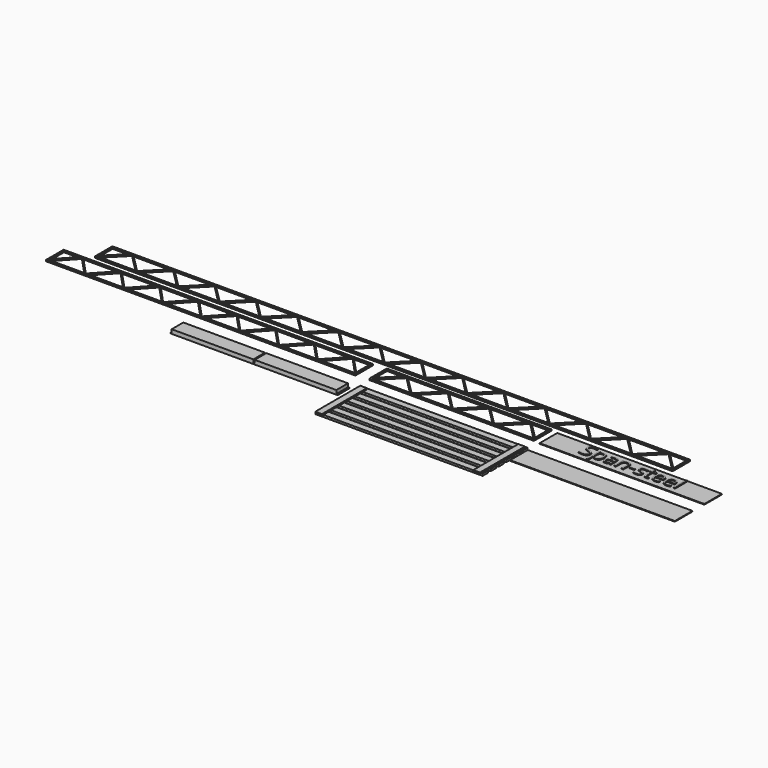
from build123d import *

# Parameters (mm, degrees)
F1_DEPTH     = 0.508
F2_W         = 63.246
F2_H         = 8.4328
F3_DEPTH     = 0.508
F5_DEPTH     = 0.508
F6_W         = 63.246
F6_H         = 8.4328
F6_W_2       = 1.8878322943
F6_H_2       = 0.5845634549
F6_W_3       = 0.6387124907
F6_H_3       = 5.9846991182
F6_TEXT_SIZE = 7.8762233922
F7_DEPTH     = 0.254
F8_DEPTH     = 0.508
F9_W         = 2.54
F9_H         = 1.905
F10_DEPTH    = 0.762
F9_W_2       = 58.166
F9_H_2       = 2.54
F9_W_3       = 0.508
F9_H_3       = 1.27
F9_H_4       = 0.635
F11_DEPTH    = 0.508
F12_W        = 0.508
F12_H        = 5.588
F12_W_2      = 31.369
F13_DEPTH    = 0.254
F14_DEPTH    = 1.58496


# Not quite as in the source:
# - Text() gives the source's letters only with a copy of the font that has no kerning and outlines rounded to 1/6400 em; it was checked with that copy


with BuildPart() as f1:
    # F0 (on Top) → F1 (new body)
    with BuildSketch(Plane.XY):
        Polygon((-113.8428, 0), (-2.8956, 0), (108.0516, 0), (108.0516, 8.4328), (-2.8956, 8.4328), (-113.8428, 8.4328), align=None)
        Polygon((-113.3348, 1.016), (-113.3348, 7.9248), (-106.426, 7.9248), align=None, mode=Mode.SUBTRACT)
        Polygon((-98.5012, 0.508), (-113.3348, 0.508), (-105.918, 7.9248), align=None, mode=Mode.SUBTRACT)
        Polygon((-90.5764, 7.9248), (-97.9932, 0.508), (-105.41, 7.9248), align=None, mode=Mode.SUBTRACT)
        Polygon((-82.6516, 0.508), (-97.4852, 0.508), (-90.0684, 7.9248), align=None, mode=Mode.SUBTRACT)
        Polygon((-74.7268, 7.9248), (-82.1436, 0.508), (-89.5604, 7.9248), align=None, mode=Mode.SUBTRACT)
        Polygon((-66.802, 0.508), (-81.6356, 0.508), (-74.2188, 7.9248), align=None, mode=Mode.SUBTRACT)
        Polygon((-58.8772, 7.9248), (-66.294, 0.508), (-73.7108, 7.9248), align=None, mode=Mode.SUBTRACT)
        Polygon((-50.9524, 0.508), (-65.786, 0.508), (-58.3692, 7.9248), align=None, mode=Mode.SUBTRACT)
        Polygon((-43.0276, 7.9248), (-50.4444, 0.508), (-57.8612, 7.9248), align=None, mode=Mode.SUBTRACT)
        Polygon((-35.1028, 0.508), (-49.9364, 0.508), (-42.5196, 7.9248), align=None, mode=Mode.SUBTRACT)
        Polygon((-27.178, 7.9248), (-34.5948, 0.508), (-42.0116, 7.9248), align=None, mode=Mode.SUBTRACT)
        Polygon((-19.2532, 0.508), (-34.0868, 0.508), (-26.67, 7.9248), align=None, mode=Mode.SUBTRACT)
        Polygon((-11.3284, 7.9248), (-18.7452, 0.508), (-26.162, 7.9248), align=None, mode=Mode.SUBTRACT)
        Polygon((-3.4036, 0.508), (-18.2372, 0.508), (-10.8204, 7.9248), align=None, mode=Mode.SUBTRACT)
        Polygon((-10.3124, 7.9248), (-2.8956, 7.9248), (4.5212, 7.9248), (-2.8956, 0.508), align=None, mode=Mode.SUBTRACT)
        Polygon((5.0292, 7.9248), (12.446, 0.508), (-2.3876, 0.508), align=None, mode=Mode.SUBTRACT)
        Polygon((20.3708, 7.9248), (12.954, 0.508), (5.5372, 7.9248), align=None, mode=Mode.SUBTRACT)
        Polygon((20.8788, 7.9248), (28.2956, 0.508), (13.462, 0.508), align=None, mode=Mode.SUBTRACT)
        Polygon((21.3868, 7.9248), (36.2204, 7.9248), (28.8036, 0.508), align=None, mode=Mode.SUBTRACT)
        Polygon((36.7284, 7.9248), (44.1452, 0.508), (29.3116, 0.508), align=None, mode=Mode.SUBTRACT)
        Polygon((52.07, 7.9248), (44.6532, 0.508), (37.2364, 7.9248), align=None, mode=Mode.SUBTRACT)
        Polygon((52.578, 7.9248), (59.9948, 0.508), (45.1612, 0.508), align=None, mode=Mode.SUBTRACT)
        Polygon((67.9196, 7.9248), (60.5028, 0.508), (53.086, 7.9248), align=None, mode=Mode.SUBTRACT)
        Polygon((75.8444, 0.508), (61.0108, 0.508), (68.4276, 7.9248), align=None, mode=Mode.SUBTRACT)
        Polygon((68.9356, 7.9248), (83.7692, 7.9248), (76.3524, 0.508), align=None, mode=Mode.SUBTRACT)
        Polygon((84.2772, 7.9248), (91.694, 0.508), (76.8604, 0.508), align=None, mode=Mode.SUBTRACT)
        Polygon((84.7852, 7.9248), (99.6188, 7.9248), (92.202, 0.508), align=None, mode=Mode.SUBTRACT)
        Polygon((100.1268, 7.9248), (107.5436, 0.508), (92.71, 0.508), align=None, mode=Mode.SUBTRACT)
        Polygon((100.6348, 7.9248), (107.5436, 7.9248), (107.5436, 1.016), align=None, mode=Mode.SUBTRACT)
    extrude(amount=F1_DEPTH)


with BuildPart() as f3:
    # F2 (on Top) → F3 (new body)
    with BuildSketch(Plane.XY):
        with Locations((31.623, -6.3287943188)):
            Rectangle(F2_W, F2_H)
        Polygon((0.508, -9.5291943188), (0.508, -2.6203943188), (7.4168, -2.6203943188), align=None, mode=Mode.SUBTRACT)
        Polygon((15.3416, -10.0371943188), (0.508, -10.0371943188), (7.9248, -2.6203943188), align=None, mode=Mode.SUBTRACT)
        Polygon((23.2664, -2.6203943188), (15.8496, -10.0371943188), (8.4328, -2.6203943188), align=None, mode=Mode.SUBTRACT)
        Polygon((31.1912, -10.0371943188), (16.3576, -10.0371943188), (23.7744, -2.6203943188), align=None, mode=Mode.SUBTRACT)
        Polygon((39.116, -2.6203943188), (31.6992, -10.0371943188), (24.2824, -2.6203943188), align=None, mode=Mode.SUBTRACT)
        Polygon((47.0408, -10.0371943188), (32.2072, -10.0371943188), (39.624, -2.6203943188), align=None, mode=Mode.SUBTRACT)
        Polygon((47.5488, -10.0371943188), (40.132, -2.6203943188), (54.9656, -2.6203943188), align=None, mode=Mode.SUBTRACT)
        Polygon((62.738, -10.0371943188), (48.0568, -10.0371943188), (55.4736, -2.6203943188), align=None, mode=Mode.SUBTRACT)
        Polygon((55.9816, -2.6203943188), (62.738, -2.6203943188), (62.738, -9.3767943188), align=None, mode=Mode.SUBTRACT)
    extrude(amount=F3_DEPTH)


with BuildPart() as f5:
    # F4 (on Top) → F5 (new body)
    with BuildSketch(Plane.XY):
        Polygon((-5.08, -10.8726160142), (-5.08, -2.4398160142), (-123.3604462539, -2.4398160142), (-123.8684462539, -2.4398160142), (-123.8684462539, -10.8726160142), (-123.3604462539, -10.8726160142), align=None)
        Polygon((-116.444168363, -2.9478160142), (-109.5278904721, -10.3646160142), (-123.3604462539, -10.3646160142), align=None, mode=Mode.SUBTRACT)
        Polygon((-101.5956125813, -2.9478160142), (-94.6793346904, -10.3646160142), (-108.5118904721, -10.3646160142), align=None, mode=Mode.SUBTRACT)
        Polygon((-86.7470567995, -2.9478160142), (-79.8307789087, -10.3646160142), (-93.6633346904, -10.3646160142), align=None, mode=Mode.SUBTRACT)
        Polygon((-57.0499452361, -2.9478160142), (-50.1336673452, -10.3646160142), (-63.9662231269, -10.3646160142), align=None, mode=Mode.SUBTRACT)
        Polygon((-42.2013894543, -2.9478160142), (-35.2851115635, -10.3646160142), (-49.1176673452, -10.3646160142), align=None, mode=Mode.SUBTRACT)
        Polygon((-116.9555484155, -2.9478160142), (-123.3604462539, -9.8195863482), (-123.3604462539, -2.9478160142), align=None, mode=Mode.SUBTRACT)
        Polygon((-108.4620648578, -9.7664212797), (-109.0198904721, -10.3646160142), (-115.9327883105, -2.9478160142), (-102.1069926338, -2.9478160142), align=None, mode=Mode.SUBTRACT)
        Polygon((-87.258436852, -2.9478160142), (-94.1713346904, -10.3646160142), (-94.7291603047, -9.7664212797), (-101.0842325287, -2.9478160142), align=None, mode=Mode.SUBTRACT)
        Polygon((-86.235676747, -2.9478160142), (-72.4098810703, -2.9478160142), (-79.3227789087, -10.3646160142), align=None, mode=Mode.SUBTRACT)
        Polygon((-71.8985010178, -2.9478160142), (-64.9822231269, -10.3646160142), (-78.8147789087, -10.3646160142), align=None, mode=Mode.SUBTRACT)
        Polygon((-57.5613252886, -2.9478160142), (-64.4742231269, -10.3646160142), (-71.3871209653, -2.9478160142), align=None, mode=Mode.SUBTRACT)
        Polygon((-56.5385651835, -2.9478160142), (-42.7127695068, -2.9478160142), (-49.0678417309, -9.7664212797), (-49.6256673452, -10.3646160142), align=None, mode=Mode.SUBTRACT)
        Polygon((-41.6900094018, -2.9478160142), (-27.8642137251, -2.9478160142), (-34.7771115635, -10.3646160142), (-35.3349371778, -9.7664212797), align=None, mode=Mode.SUBTRACT)
        Polygon((-27.3528336726, -2.9478160142), (-20.4365557817, -10.3646160142), (-34.2691115635, -10.3646160142), align=None, mode=Mode.SUBTRACT)
        Polygon((-26.8414536201, -2.9478160142), (-13.0156579434, -2.9478160142), (-19.3707301674, -9.7664212797), (-19.9285557817, -10.3646160142), align=None, mode=Mode.SUBTRACT)
        Polygon((-12.5042778909, -2.9478160142), (-5.588, -10.3646160142), (-19.4205557817, -10.3646160142), align=None, mode=Mode.SUBTRACT)
        Polygon((-11.9928978384, -2.9478160142), (-5.588, -2.9478160142), (-5.588, -9.8566160142), align=None, mode=Mode.SUBTRACT)
    extrude(amount=F5_DEPTH)


with BuildPart() as f7:
    # F6 (on Top) → F7 (new body)
    with BuildSketch(Plane.XY):
        with Locations((97.409, -6.7564)):
            Rectangle(F6_W, F6_H)
        with BuildLine():
            add(Edge.make_bspline(
                [(81.9722174812, -6.2846355502), (82.3044956555, -6.6464495623), (82.3044956555, -7.2223983979)],
                knots=[0, 0, 0, 1, 1, 1], degree=2))
            add(Edge.make_bspline(
                [(82.3044956555, -7.2223983979), (82.3044956555, -7.9644863206), (81.7660819471, -8.3804493685)],
                knots=[0, 0, 0, 1, 1, 1], degree=2))
            add(Edge.make_bspline(
                [(81.7660819471, -8.3804493685), (81.2276682386, -8.7964124164), (80.3046733099, -8.7964124164)],
                knots=[0, 0, 0, 1, 1, 1], degree=2))
            add(Edge.make_bspline(
                [(80.3046733099, -8.7964124164), (79.305377467, -8.7964124164), (78.7663484286, -8.5379738364)],
                knots=[0, 0, 0, 1, 1, 1], degree=2))
            Line((78.7663484286, -8.5379738364), (78.7663484286, -7.907875965))
            add(Edge.make_bspline(
                [(78.7663484286, -7.907875965), (79.1133945218, -8.0530938338), (79.5207429504, -8.1380093672)],
                knots=[0, 0, 0, 1, 1, 1], degree=2))
            add(Edge.make_bspline(
                [(79.5207429504, -8.1380093672), (79.9280913789, -8.2229249007), (80.3280558481, -8.2229249007)],
                knots=[0, 0, 0, 1, 1, 1], degree=2))
            add(Edge.make_bspline(
                [(80.3280558481, -8.2229249007), (80.9815362576, -8.2229249007), (81.3125837721, -7.9749469298)],
                knots=[0, 0, 0, 1, 1, 1], degree=2))
            add(Edge.make_bspline(
                [(81.3125837721, -7.9749469298), (81.6436312865, -7.7269689589), (81.6436312865, -7.2839313931)],
                knots=[0, 0, 0, 1, 1, 1], degree=2))
            add(Edge.make_bspline(
                [(81.6436312865, -7.2839313931), (81.6436312865, -6.9922649956), (81.5261032656, -6.80582002)],
                knots=[0, 0, 0, 1, 1, 1], degree=2))
            add(Edge.make_bspline(
                [(81.5261032656, -6.80582002), (81.4085752447, -6.6193750444), (81.1335227559, -6.4612352466)],
                knots=[0, 0, 0, 1, 1, 1], degree=2))
            add(Edge.make_bspline(
                [(81.1335227559, -6.4612352466), (80.8584702671, -6.3030954488), (80.2972893504, -6.1037285442)],
                knots=[0, 0, 0, 1, 1, 1], degree=2))
            add(Edge.make_bspline(
                [(80.2972893504, -6.1037285442), (79.5133589909, -5.8231380859), (79.1767735069, -5.4385568655)],
                knots=[0, 0, 0, 1, 1, 1], degree=2))
            add(Edge.make_bspline(
                [(79.1767735069, -5.4385568655), (78.8401880229, -5.0539756452), (78.8401880229, -4.434953713)],
                knots=[0, 0, 0, 1, 1, 1], degree=2))
            add(Edge.make_bspline(
                [(78.8401880229, -4.434953713), (78.8401880229, -3.7851652831), (79.3281446752, -3.4005840628)],
                knots=[0, 0, 0, 1, 1, 1], degree=2))
            add(Edge.make_bspline(
                [(79.3281446752, -3.4005840628), (79.8161013276, -3.0160028425), (80.6209529055, -3.0160028425)],
                knots=[0, 0, 0, 1, 1, 1], degree=2))
            add(Edge.make_bspline(
                [(80.6209529055, -3.0160028425), (81.4590323008, -3.0160028425), (82.1629697665, -3.3236678187)],
                knots=[0, 0, 0, 1, 1, 1], degree=2))
            Line((82.1629697665, -3.3236678187), (81.9586802222, -3.8922326949))
            add(Edge.make_bspline(
                [(81.9586802222, -3.8922326949), (81.262126716, -3.6005662974), (80.6049543267, -3.6005662974)],
                knots=[0, 0, 0, 1, 1, 1], degree=2))
            add(Edge.make_bspline(
                [(80.6049543267, -3.6005662974), (80.0856158468, -3.6005662974), (79.7933341193, -3.8233157402)],
                knots=[0, 0, 0, 1, 1, 1], degree=2))
            add(Edge.make_bspline(
                [(79.7933341193, -3.8233157402), (79.5010523919, -4.046065183), (79.5010523919, -4.4423376724)],
                knots=[0, 0, 0, 1, 1, 1], degree=2))
            add(Edge.make_bspline(
                [(79.5010523919, -4.4423376724), (79.5010523919, -4.7340040699), (79.6087351336, -4.9210643755)],
                knots=[0, 0, 0, 1, 1, 1], degree=2))
            add(Edge.make_bspline(
                [(79.6087351336, -4.9210643755), (79.7164178753, -5.108124681), (79.9723951355, -5.263803159)],
                knots=[0, 0, 0, 1, 1, 1], degree=2))
            add(Edge.make_bspline(
                [(79.9723951355, -5.263803159), (80.2283723957, -5.419481637), (80.7550948351, -5.6077726025)],
                knots=[0, 0, 0, 1, 1, 1], degree=2))
            add(Edge.make_bspline(
                [(80.7550948351, -5.6077726025), (81.6399393068, -5.9228215382), (81.9722174812, -6.2846355502)],
                knots=[0, 0, 0, 1, 1, 1], degree=2))
        make_face(mode=Mode.SUBTRACT)
        with BuildLine():
            add(Edge.make_bspline(
                [(86.6074980135, -8.2210789108), (86.1441545593, -8.7964124164), (85.3208430828, -8.7964124164)],
                knots=[0, 0, 0, 1, 1, 1], degree=2))
            add(Edge.make_bspline(
                [(85.3208430828, -8.7964124164), (84.9085720146, -8.7964124164), (84.5682945509, -8.6444259181)],
                knots=[0, 0, 0, 1, 1, 1], degree=2))
            add(Edge.make_bspline(
                [(84.5682945509, -8.6444259181), (84.2280170871, -8.4924394199), (83.9978836849, -8.1761598243)],
                knots=[0, 0, 0, 1, 1, 1], degree=2))
            Line((83.9978836849, -8.1761598243), (83.9511186085, -8.1761598243))
            add(Edge.make_bspline(
                [(83.9511186085, -8.1761598243), (83.9978836849, -8.5453577958), (83.9978836849, -8.8764053102)],
                knots=[0, 0, 0, 1, 1, 1], degree=2))
            Line((83.9978836849, -8.8764053102), (83.9978836849, -10.6116357763))
            Line((83.9978836849, -10.6116357763), (83.3591711942, -10.6116357763))
            Line((83.3591711942, -10.6116357763), (83.3591711942, -4.5038706677))
            Line((83.3591711942, -4.5038706677), (83.8785096741, -4.5038706677))
            Line((83.8785096741, -4.5038706677), (83.9671171872, -5.0810501631))
            Line((83.9671171872, -5.0810501631), (83.9978836849, -5.0810501631))
            add(Edge.make_bspline(
                [(83.9978836849, -5.0810501631), (84.2440156659, -4.7340040699), (84.5707558707, -4.5801715818)],
                knots=[0, 0, 0, 1, 1, 1], degree=2))
            add(Edge.make_bspline(
                [(84.5707558707, -4.5801715818), (84.8974960755, -4.4263390936), (85.3208430828, -4.4263390936)],
                knots=[0, 0, 0, 1, 1, 1], degree=2))
            add(Edge.make_bspline(
                [(85.3208430828, -4.4263390936), (86.1589224781, -4.4263390936), (86.6148819729, -4.9998266094)],
                knots=[0, 0, 0, 1, 1, 1], degree=2))
            add(Edge.make_bspline(
                [(86.6148819729, -4.9998266094), (87.0708414677, -5.5733141251), (87.0708414677, -6.6070684454)],
                knots=[0, 0, 0, 1, 1, 1], degree=2))
            add(Edge.make_bspline(
                [(87.0708414677, -6.6070684454), (87.0708414677, -7.6457454052), (86.6074980135, -8.2210789108)],
                knots=[0, 0, 0, 1, 1, 1], degree=2))
        make_face(mode=Mode.SUBTRACT)
        with BuildLine():
            Line((91.2513931652, -8.7188808424), (90.7775891017, -8.7188808424))
            Line((90.7775891017, -8.7188808424), (90.6508311315, -8.1183188087))
            Line((90.6508311315, -8.1183188087), (90.6200646339, -8.1183188087))
            add(Edge.make_bspline(
                [(90.6200646339, -8.1183188087), (90.3050156982, -8.5145912982), (89.9918127523, -8.6555018573)],
                knots=[0, 0, 0, 1, 1, 1], degree=2))
            add(Edge.make_bspline(
                [(89.9918127523, -8.6555018573), (89.6786098065, -8.7964124164), (89.2084977228, -8.7964124164)],
                knots=[0, 0, 0, 1, 1, 1], degree=2))
            add(Edge.make_bspline(
                [(89.2084977228, -8.7964124164), (88.5820918311, -8.7964124164), (88.2264311186, -8.4727488614)],
                knots=[0, 0, 0, 1, 1, 1], degree=2))
            add(Edge.make_bspline(
                [(88.2264311186, -8.4727488614), (87.870770406, -8.1490853064), (87.870770406, -7.5534459123)],
                knots=[0, 0, 0, 1, 1, 1], degree=2))
            add(Edge.make_bspline(
                [(87.870770406, -7.5534459123), (87.870770406, -6.2772515908), (89.9124351885, -6.2157185956)],
                knots=[0, 0, 0, 1, 1, 1], degree=2))
            Line((89.9124351885, -6.2157185956), (90.6274485933, -6.1923360574))
            Line((90.6274485933, -6.1923360574), (90.6274485933, -5.9302054976))
            add(Edge.make_bspline(
                [(90.6274485933, -5.9302054976), (90.6274485933, -5.4342495559), (90.4145444297, -5.1979628541)],
                knots=[0, 0, 0, 1, 1, 1], degree=2))
            add(Edge.make_bspline(
                [(90.4145444297, -5.1979628541), (90.2016402662, -4.9616761523), (89.7315281824, -4.9616761523)],
                knots=[0, 0, 0, 1, 1, 1], degree=2))
            add(Edge.make_bspline(
                [(89.7315281824, -4.9616761523), (89.2048057431, -4.9616761523), (88.5402493944, -5.2841090474)],
                knots=[0, 0, 0, 1, 1, 1], degree=2))
            Line((88.5402493944, -5.2841090474), (88.3433438096, -4.7955370652))
            add(Edge.make_bspline(
                [(88.3433438096, -4.7955370652), (88.6547007655, -4.6269366582), (89.0257447269, -4.5309451856)],
                knots=[0, 0, 0, 1, 1, 1], degree=2))
            add(Edge.make_bspline(
                [(89.0257447269, -4.5309451856), (89.3967886883, -4.434953713), (89.7709092994, -4.434953713)],
                knots=[0, 0, 0, 1, 1, 1], degree=2))
            add(Edge.make_bspline(
                [(89.7709092994, -4.434953713), (90.5240731613, -4.434953713), (90.8877331632, -4.7690778772)],
                knots=[0, 0, 0, 1, 1, 1], degree=2))
            add(Edge.make_bspline(
                [(90.8877331632, -4.7690778772), (91.2513931652, -5.1032020414), (91.2513931652, -5.8415979844)],
                knots=[0, 0, 0, 1, 1, 1], degree=2))
            Line((91.2513931652, -5.8415979844), (91.2513931652, -8.7188808424))
        make_face(mode=Mode.SUBTRACT)
        with BuildLine():
            Line((96.0891172518, -8.7188808424), (95.4504047611, -8.7188808424))
            Line((95.4504047611, -8.7188808424), (95.4504047611, -5.9917384928))
            add(Edge.make_bspline(
                [(95.4504047611, -5.9917384928), (95.4504047611, -5.4773226525), (95.2159640492, -5.2231913822)],
                knots=[0, 0, 0, 1, 1, 1], degree=2))
            add(Edge.make_bspline(
                [(95.2159640492, -5.2231913822), (94.9815233373, -4.9690601118), (94.480644756, -4.9690601118)],
                knots=[0, 0, 0, 1, 1, 1], degree=2))
            add(Edge.make_bspline(
                [(94.480644756, -4.9690601118), (93.819780387, -4.9690601118), (93.5121154107, -5.3265668142)],
                knots=[0, 0, 0, 1, 1, 1], degree=2))
            add(Edge.make_bspline(
                [(93.5121154107, -5.3265668142), (93.2044504344, -5.6840735166), (93.2044504344, -6.5073849931)],
                knots=[0, 0, 0, 1, 1, 1], degree=2))
            Line((93.2044504344, -6.5073849931), (93.2044504344, -8.7188808424))
            Line((93.2044504344, -8.7188808424), (92.5657379437, -8.7188808424))
            Line((92.5657379437, -8.7188808424), (92.5657379437, -4.5038706677))
            Line((92.5657379437, -4.5038706677), (93.0850764237, -4.5038706677))
            Line((93.0850764237, -4.5038706677), (93.1884518557, -5.0810501631))
            Line((93.1884518557, -5.0810501631), (93.2192183533, -5.0810501631))
            add(Edge.make_bspline(
                [(93.2192183533, -5.0810501631), (93.4161239381, -4.7696932071), (93.7699386608, -4.5980161504)],
                knots=[0, 0, 0, 1, 1, 1], degree=2))
            add(Edge.make_bspline(
                [(93.7699386608, -4.5980161504), (94.1237533835, -4.4263390936), (94.55817633, -4.4263390936)],
                knots=[0, 0, 0, 1, 1, 1], degree=2))
            add(Edge.make_bspline(
                [(94.55817633, -4.4263390936), (95.3199548112, -4.4263390936), (95.7045360315, -4.7936910753)],
                knots=[0, 0, 0, 1, 1, 1], degree=2))
            add(Edge.make_bspline(
                [(95.7045360315, -4.7936910753), (96.0891172518, -5.1610430569), (96.0891172518, -5.9695866146)],
                knots=[0, 0, 0, 1, 1, 1], degree=2))
            Line((96.0891172518, -5.9695866146), (96.0891172518, -8.7188808424))
        make_face(mode=Mode.SUBTRACT)
        with Locations((97.9904868051, -6.6076837753)):
            Rectangle(F6_W_2, F6_H_2, mode=Mode.SUBTRACT)
        with BuildLine():
            add(Edge.make_bspline(
                [(102.3888653057, -6.8728909849), (102.6522265254, -7.1497894635), (102.6522265254, -7.5694444911)],
                knots=[0, 0, 0, 1, 1, 1], degree=2))
            add(Edge.make_bspline(
                [(102.6522265254, -7.5694444911), (102.6522265254, -8.1576999257), (102.2141115992, -8.4770561711)],
                knots=[0, 0, 0, 1, 1, 1], degree=2))
            add(Edge.make_bspline(
                [(102.2141115992, -8.4770561711), (101.775996673, -8.7964124164), (100.9834516942, -8.7964124164)],
                knots=[0, 0, 0, 1, 1, 1], degree=2))
            add(Edge.make_bspline(
                [(100.9834516942, -8.7964124164), (100.1453722988, -8.7964124164), (99.676490875, -8.5305898769)],
                knots=[0, 0, 0, 1, 1, 1], degree=2))
            Line((99.676490875, -8.5305898769), (99.676490875, -7.9386424626))
            add(Edge.make_bspline(
                [(99.676490875, -7.9386424626), (99.9804638716, -8.0924749507), (100.3281252947, -8.180467134)],
                knots=[0, 0, 0, 1, 1, 1], degree=2))
            add(Edge.make_bspline(
                [(100.3281252947, -8.180467134), (100.6757867179, -8.2684593172), (100.9994502729, -8.2684593172)],
                knots=[0, 0, 0, 1, 1, 1], degree=2))
            add(Edge.make_bspline(
                [(100.9994502729, -8.2684593172), (101.4990981944, -8.2684593172), (101.7679973836, -8.1090888595)],
                knots=[0, 0, 0, 1, 1, 1], degree=2))
            add(Edge.make_bspline(
                [(101.7679973836, -8.1090888595), (102.0368965729, -7.9497184018), (102.0368965729, -7.622362867)],
                knots=[0, 0, 0, 1, 1, 1], degree=2))
            add(Edge.make_bspline(
                [(102.0368965729, -7.622362867), (102.0368965729, -7.376230886), (101.8239924093, -7.2014771795)],
                knots=[0, 0, 0, 1, 1, 1], degree=2))
            add(Edge.make_bspline(
                [(101.8239924093, -7.2014771795), (101.6110882457, -7.026723473), (100.9908356536, -6.7879754514)],
                knots=[0, 0, 0, 1, 1, 1], degree=2))
            add(Edge.make_bspline(
                [(100.9908356536, -6.7879754514), (100.402580219, -6.5689179883), (100.1546022481, -6.4052402209)],
                knots=[0, 0, 0, 1, 1, 1], degree=2))
            add(Edge.make_bspline(
                [(100.1546022481, -6.4052402209), (99.9066242773, -6.2415624536), (99.7854042766, -6.0341962596)],
                knots=[0, 0, 0, 1, 1, 1], degree=2))
            add(Edge.make_bspline(
                [(99.7854042766, -6.0341962596), (99.664184276, -5.8268300656), (99.664184276, -5.5388556478)],
                knots=[0, 0, 0, 1, 1, 1], degree=2))
            add(Edge.make_bspline(
                [(99.664184276, -5.5388556478), (99.664184276, -5.0232091476), (100.0838393036, -4.7247741206)],
                knots=[0, 0, 0, 1, 1, 1], degree=2))
            add(Edge.make_bspline(
                [(100.0838393036, -4.7247741206), (100.5034943312, -4.4263390936), (101.2332756549, -4.4263390936)],
                knots=[0, 0, 0, 1, 1, 1], degree=2))
            add(Edge.make_bspline(
                [(101.2332756549, -4.4263390936), (101.9138305824, -4.4263390936), (102.5648496721, -4.7032375723)],
                knots=[0, 0, 0, 1, 1, 1], degree=2))
            Line((102.5648496721, -4.7032375723), (102.3371775897, -5.2225760522))
            add(Edge.make_bspline(
                [(102.3371775897, -5.2225760522), (101.7033877386, -4.9616761523), (101.1877412384, -4.9616761523)],
                knots=[0, 0, 0, 1, 1, 1], degree=2))
            add(Edge.make_bspline(
                [(101.1877412384, -4.9616761523), (100.7336277335, -4.9616761523), (100.5028790013, -5.1038173714)],
                knots=[0, 0, 0, 1, 1, 1], degree=2))
            add(Edge.make_bspline(
                [(100.5028790013, -5.1038173714), (100.2721302691, -5.2459585904), (100.2721302691, -5.4957825511)],
                knots=[0, 0, 0, 1, 1, 1], degree=2))
            add(Edge.make_bspline(
                [(100.2721302691, -5.4957825511), (100.2721302691, -5.665613618), (100.3588917924, -5.7843722988)],
                knots=[0, 0, 0, 1, 1, 1], degree=2))
            add(Edge.make_bspline(
                [(100.3588917924, -5.7843722988), (100.4456533157, -5.9031309797), (100.6376362609, -6.0108137214)],
                knots=[0, 0, 0, 1, 1, 1], degree=2))
            add(Edge.make_bspline(
                [(100.6376362609, -6.0108137214), (100.829619206, -6.1184964631), (101.3760322039, -6.3227860073)],
                knots=[0, 0, 0, 1, 1, 1], degree=2))
            add(Edge.make_bspline(
                [(101.3760322039, -6.3227860073), (102.125504086, -6.5959925062), (102.3888653057, -6.8728909849)],
                knots=[0, 0, 0, 1, 1, 1], degree=2))
        make_face(mode=Mode.SUBTRACT)
        with BuildLine():
            add(Edge.make_bspline(
                [(104.5560573985, -8.0647851029), (104.7369644045, -8.2684593172), (105.0520133402, -8.2684593172)],
                knots=[0, 0, 0, 1, 1, 1], degree=2))
            add(Edge.make_bspline(
                [(105.0520133402, -8.2684593172), (105.2218444071, -8.2684593172), (105.379368875, -8.2438461191)],
                knots=[0, 0, 0, 1, 1, 1], degree=2))
            add(Edge.make_bspline(
                [(105.379368875, -8.2438461191), (105.5368933428, -8.219232921), (105.6291928357, -8.192158403)],
                knots=[0, 0, 0, 1, 1, 1], degree=2))
            Line((105.6291928357, -8.192158403), (105.6291928357, -8.6807303853))
            add(Edge.make_bspline(
                [(105.6291928357, -8.6807303853), (105.5258174037, -8.7299567815), (105.3239891792, -8.763184599)],
                knots=[0, 0, 0, 1, 1, 1], degree=2))
            add(Edge.make_bspline(
                [(105.3239891792, -8.763184599), (105.1221609548, -8.7964124164), (104.9597138473, -8.7964124164)],
                knots=[0, 0, 0, 1, 1, 1], degree=2))
            add(Edge.make_bspline(
                [(104.9597138473, -8.7964124164), (103.7376685616, -8.7964124164), (103.7376685616, -7.5079114958)],
                knots=[0, 0, 0, 1, 1, 1], degree=2))
            Line((103.7376685616, -7.5079114958), (103.7376685616, -4.9998266094))
            Line((103.7376685616, -4.9998266094), (103.1334145483, -4.9998266094))
            Line((103.1334145483, -4.9998266094), (103.1334145483, -4.6921616331))
            Line((103.1334145483, -4.6921616331), (103.7376685616, -4.4263390936))
            Line((103.7376685616, -4.4263390936), (104.0059524209, -3.5267267031))
            Line((104.0059524209, -3.5267267031), (104.3751503925, -3.5267267031))
            Line((104.3751503925, -3.5267267031), (104.3751503925, -4.5038706677))
            Line((104.3751503925, -4.5038706677), (105.5984263381, -4.5038706677))
            Line((105.5984263381, -4.5038706677), (105.5984263381, -4.9998266094))
            Line((105.5984263381, -4.9998266094), (104.3751503925, -4.9998266094))
            Line((104.3751503925, -4.9998266094), (104.3751503925, -7.4808369779))
            add(Edge.make_bspline(
                [(104.3751503925, -7.4808369779), (104.3751503925, -7.8611108886), (104.5560573985, -8.0647851029)],
                knots=[0, 0, 0, 1, 1, 1], degree=2))
        make_face(mode=Mode.SUBTRACT)
        with BuildLine():
            add(Edge.make_bspline(
                [(108.9802797571, -8.7324181014), (108.6787680804, -8.7964124164), (108.2517290933, -8.7964124164)],
                knots=[0, 0, 0, 1, 1, 1], degree=2))
            add(Edge.make_bspline(
                [(108.2517290933, -8.7964124164), (107.3176582254, -8.7964124164), (106.7767831971, -8.2266168804)],
                knots=[0, 0, 0, 1, 1, 1], degree=2))
            add(Edge.make_bspline(
                [(106.7767831971, -8.2266168804), (106.2359081689, -7.6568213444), (106.2359081689, -6.6464495623)],
                knots=[0, 0, 0, 1, 1, 1], degree=2))
            add(Edge.make_bspline(
                [(106.2359081689, -6.6464495623), (106.2359081689, -5.626232501), (106.7380174101, -5.0262857973)],
                knots=[0, 0, 0, 1, 1, 1], degree=2))
            add(Edge.make_bspline(
                [(106.7380174101, -5.0262857973), (107.2401266514, -4.4263390936), (108.086820666, -4.4263390936)],
                knots=[0, 0, 0, 1, 1, 1], degree=2))
            add(Edge.make_bspline(
                [(108.086820666, -4.4263390936), (108.878134985, -4.4263390936), (109.3396324494, -4.9475235634)],
                knots=[0, 0, 0, 1, 1, 1], degree=2))
            add(Edge.make_bspline(
                [(109.3396324494, -4.9475235634), (109.8011299138, -5.4687080332), (109.8011299138, -6.3227860073)],
                knots=[0, 0, 0, 1, 1, 1], degree=2))
            Line((109.8011299138, -6.3227860073), (109.8011299138, -6.7264424562))
            Line((109.8011299138, -6.7264424562), (106.8980031978, -6.7264424562))
            add(Edge.make_bspline(
                [(106.8980031978, -6.7264424562), (106.9176937563, -7.4685303789), (107.2733544688, -7.8531115992)],
                knots=[0, 0, 0, 1, 1, 1], degree=2))
            add(Edge.make_bspline(
                [(107.2733544688, -7.8531115992), (107.6290151814, -8.2376928195), (108.2751116315, -8.2376928195)],
                knots=[0, 0, 0, 1, 1, 1], degree=2))
            add(Edge.make_bspline(
                [(108.2751116315, -8.2376928195), (108.955666559, -8.2376928195), (109.6202229077, -7.9534103815)],
                knots=[0, 0, 0, 1, 1, 1], degree=2))
            Line((109.6202229077, -7.9534103815), (109.6202229077, -8.5232059175))
            add(Edge.make_bspline(
                [(109.6202229077, -8.5232059175), (109.2817914338, -8.6684237863), (108.9802797571, -8.7324181014)],
                knots=[0, 0, 0, 1, 1, 1], degree=2))
        make_face(mode=Mode.SUBTRACT)
        with BuildLine():
            add(Edge.make_bspline(
                [(113.3995794761, -8.7324181014), (113.0980677993, -8.7964124164), (112.6710288123, -8.7964124164)],
                knots=[0, 0, 0, 1, 1, 1], degree=2))
            add(Edge.make_bspline(
                [(112.6710288123, -8.7964124164), (111.7369579444, -8.7964124164), (111.1960829161, -8.2266168804)],
                knots=[0, 0, 0, 1, 1, 1], degree=2))
            add(Edge.make_bspline(
                [(111.1960829161, -8.2266168804), (110.6552078879, -7.6568213444), (110.6552078879, -6.6464495623)],
                knots=[0, 0, 0, 1, 1, 1], degree=2))
            add(Edge.make_bspline(
                [(110.6552078879, -6.6464495623), (110.6552078879, -5.626232501), (111.1573171291, -5.0262857973)],
                knots=[0, 0, 0, 1, 1, 1], degree=2))
            add(Edge.make_bspline(
                [(111.1573171291, -5.0262857973), (111.6594263704, -4.4263390936), (112.506120385, -4.4263390936)],
                knots=[0, 0, 0, 1, 1, 1], degree=2))
            add(Edge.make_bspline(
                [(112.506120385, -4.4263390936), (113.297434704, -4.4263390936), (113.7589321684, -4.9475235634)],
                knots=[0, 0, 0, 1, 1, 1], degree=2))
            add(Edge.make_bspline(
                [(113.7589321684, -4.9475235634), (114.2204296327, -5.4687080332), (114.2204296327, -6.3227860073)],
                knots=[0, 0, 0, 1, 1, 1], degree=2))
            Line((114.2204296327, -6.3227860073), (114.2204296327, -6.7264424562))
            Line((114.2204296327, -6.7264424562), (111.3173029168, -6.7264424562))
            add(Edge.make_bspline(
                [(111.3173029168, -6.7264424562), (111.3369934752, -7.4685303789), (111.6926541878, -7.8531115992)],
                knots=[0, 0, 0, 1, 1, 1], degree=2))
            add(Edge.make_bspline(
                [(111.6926541878, -7.8531115992), (112.0483149004, -8.2376928195), (112.6944113505, -8.2376928195)],
                knots=[0, 0, 0, 1, 1, 1], degree=2))
            add(Edge.make_bspline(
                [(112.6944113505, -8.2376928195), (113.374966278, -8.2376928195), (114.0395226267, -7.9534103815)],
                knots=[0, 0, 0, 1, 1, 1], degree=2))
            Line((114.0395226267, -7.9534103815), (114.0395226267, -8.5232059175))
            add(Edge.make_bspline(
                [(114.0395226267, -8.5232059175), (113.7010911528, -8.6684237863), (113.3995794761, -8.7324181014)],
                knots=[0, 0, 0, 1, 1, 1], degree=2))
        make_face(mode=Mode.SUBTRACT)
        with Locations((115.6289198941, -5.7265312833)):
            Rectangle(F6_W_3, F6_H_3, mode=Mode.SUBTRACT)
        with Locations((97.409, -20.9161403965)):
            Rectangle(F6_W, F6_H)
        with BuildLine():
            add(Edge.make_bspline(
                [(86.0992354727, -5.3899457993), (85.7897245066, -4.9690601118), (85.2285435899, -4.9690601118)],
                knots=[0, 0, 0, 1, 1, 1], degree=2))
            add(Edge.make_bspline(
                [(85.2285435899, -4.9690601118), (84.5824471398, -4.9690601118), (84.293857392, -5.3265668142)],
                knots=[0, 0, 0, 1, 1, 1], degree=2))
            add(Edge.make_bspline(
                [(84.293857392, -5.3265668142), (84.0052676443, -5.6840735166), (83.9978836849, -6.4655425563)],
                knots=[0, 0, 0, 1, 1, 1], degree=2))
            Line((83.9978836849, -6.4655425563), (83.9978836849, -6.6070684454))
            add(Edge.make_bspline(
                [(83.9978836849, -6.6070684454), (83.9978836849, -7.4956048968), (84.293857392, -7.8783401273)],
                knots=[0, 0, 0, 1, 1, 1], degree=2))
            add(Edge.make_bspline(
                [(84.293857392, -7.8783401273), (84.5898310992, -8.2610753577), (85.2433115088, -8.2610753577)],
                knots=[0, 0, 0, 1, 1, 1], degree=2))
            add(Edge.make_bspline(
                [(85.2433115088, -8.2610753577), (85.7897245066, -8.2610753577), (86.0992354727, -7.8186531219)],
                knots=[0, 0, 0, 1, 1, 1], degree=2))
            add(Edge.make_bspline(
                [(86.0992354727, -7.8186531219), (86.4087464388, -7.376230886), (86.4087464388, -6.5996844859)],
                knots=[0, 0, 0, 1, 1, 1], degree=2))
            add(Edge.make_bspline(
                [(86.4087464388, -6.5996844859), (86.4087464388, -5.8108314868), (86.0992354727, -5.3899457993)],
                knots=[0, 0, 0, 1, 1, 1], degree=2))
        make_face()
        with BuildLine():
            add(Edge.make_bspline(
                [(88.7494615782, -8.0881676411), (88.9586737621, -8.2684593172), (89.335255693, -8.2684593172)],
                knots=[0, 0, 0, 1, 1, 1], degree=2))
            add(Edge.make_bspline(
                [(89.335255693, -8.2684593172), (89.932125747, -8.2684593172), (90.2724032107, -7.9417191124)],
                knots=[0, 0, 0, 1, 1, 1], degree=2))
            add(Edge.make_bspline(
                [(90.2724032107, -7.9417191124), (90.6126806744, -7.6149789076), (90.6126806744, -7.026723473)],
                knots=[0, 0, 0, 1, 1, 1], degree=2))
            Line((90.6126806744, -7.026723473), (90.6126806744, -6.6464495623))
            Line((90.6126806744, -6.6464495623), (89.9739681837, -6.6722934203))
            add(Edge.make_bspline(
                [(89.9739681837, -6.6722934203), (89.2121897025, -6.6993679382), (88.8762195484, -6.909195452)],
                knots=[0, 0, 0, 1, 1, 1], degree=2))
            add(Edge.make_bspline(
                [(88.8762195484, -6.909195452), (88.5402493944, -7.1190229659), (88.5402493944, -7.5608298718)],
                knots=[0, 0, 0, 1, 1, 1], degree=2))
            add(Edge.make_bspline(
                [(88.5402493944, -7.5608298718), (88.5402493944, -7.907875965), (88.7494615782, -8.0881676411)],
                knots=[0, 0, 0, 1, 1, 1], degree=2))
        make_face()
        with BuildLine():
            add(Edge.make_bspline(
                [(108.8479838173, -5.2828783875), (108.5790846281, -4.9616761523), (108.0782060467, -4.9616761523)],
                knots=[0, 0, 0, 1, 1, 1], degree=2))
            add(Edge.make_bspline(
                [(108.0782060467, -4.9616761523), (107.5711741658, -4.9616761523), (107.2690471591, -5.2921083368)],
                knots=[0, 0, 0, 1, 1, 1], degree=2))
            add(Edge.make_bspline(
                [(107.2690471591, -5.2921083368), (106.9669201525, -5.6225405213), (106.9127711166, -6.2071039762)],
                knots=[0, 0, 0, 1, 1, 1], degree=2))
            Line((106.9127711166, -6.2071039762), (109.1168830066, -6.2071039762))
            add(Edge.make_bspline(
                [(109.1168830066, -6.2071039762), (109.1168830066, -5.6040806228), (108.8479838173, -5.2828783875)],
                knots=[0, 0, 0, 1, 1, 1], degree=2))
        make_face()
        with BuildLine():
            add(Edge.make_bspline(
                [(113.2672835363, -5.2828783875), (112.998384347, -4.9616761523), (112.4975057657, -4.9616761523)],
                knots=[0, 0, 0, 1, 1, 1], degree=2))
            add(Edge.make_bspline(
                [(112.4975057657, -4.9616761523), (111.9904738848, -4.9616761523), (111.6883468781, -5.2921083368)],
                knots=[0, 0, 0, 1, 1, 1], degree=2))
            add(Edge.make_bspline(
                [(111.6883468781, -5.2921083368), (111.3862198714, -5.6225405213), (111.3320708356, -6.2071039762)],
                knots=[0, 0, 0, 1, 1, 1], degree=2))
            Line((111.3320708356, -6.2071039762), (113.5361827255, -6.2071039762))
            add(Edge.make_bspline(
                [(113.5361827255, -6.2071039762), (113.5361827255, -5.6040806228), (113.2672835363, -5.2828783875)],
                knots=[0, 0, 0, 1, 1, 1], degree=2))
        make_face()
        with Locations((78.359, -8.7188808424)):
            Text('Span-steel', F6_TEXT_SIZE, font='Open Sans', text_align=(TextAlign.LEFT, TextAlign.BOTTOM))
    extrude(amount=F7_DEPTH)


with BuildPart() as f8:
    # F6 (on Top) → F8 (new body)
    with BuildSketch(Plane.XY):
        with Locations((78.359, -8.7188808424)):
            Text('Span-steel', F6_TEXT_SIZE, font='Open Sans', text_align=(TextAlign.LEFT, TextAlign.BOTTOM))
    extrude(amount=F8_DEPTH)


with BuildPart() as f10:
    # F9 (on Top) → F10 (new body)
    with BuildSketch(Plane.XY):
        Polygon((64.516, -15.1895204921), (0.254, -15.1895204921), (0.254, -17.7295204921), (0.762, -17.7295204921), (0.762, -15.8245204921), (3.302, -15.8245204921), (3.302, -17.7295204921), (61.468, -17.7295204921), (61.468, -15.8245204921), (64.008, -15.8245204921), (64.008, -17.7295204921), (64.516, -17.7295204921), align=None)
        with Locations((2.032, -16.7770204921)):
            Rectangle(F9_W, F9_H)
        with Locations((62.738, -16.7770204921)):
            Rectangle(F9_W, F9_H)
    extrude(amount=-F10_DEPTH)


with BuildPart() as f10b:
    # F9 (on Top) → F10, piece 2 (new body)
    with BuildSketch(Plane.XY):
        with Locations((32.385, -20.2695204921)):
            Rectangle(F9_W_2, F9_H_2)
        with Locations((2.032, -20.2695204921)):
            Rectangle(F9_W, F9_H_2)
        with Locations((0.508, -20.2695204921)):
            Rectangle(F9_W_3, F9_H_2)
        with Locations((62.738, -20.2695204921)):
            Rectangle(F9_W, F9_H_2)
        with Locations((64.262, -20.2695204921)):
            Rectangle(F9_W_3, F9_H_2)
    extrude(amount=-F10_DEPTH)


with BuildPart() as f10c:
    # F9 (on Top) → F10, piece 3 (new body)
    with BuildSketch(Plane.XY):
        with Locations((32.385, -24.0795204921)):
            Rectangle(F9_W_2, F9_H_2)
        with Locations((2.032, -24.0795204921)):
            Rectangle(F9_W, F9_H_2)
        with Locations((0.508, -24.0795204921)):
            Rectangle(F9_W_3, F9_H_2)
        with Locations((64.262, -24.0795204921)):
            Rectangle(F9_W_3, F9_H_2)
        with Locations((62.738, -24.0795204921)):
            Rectangle(F9_W, F9_H_2)
    extrude(amount=-F10_DEPTH)


with BuildPart() as f10d:
    # F9 (on Top) → F10, piece 4 (new body)
    with BuildSketch(Plane.XY):
        with Locations((32.385, -27.8895204921)):
            Rectangle(F9_W_2, F9_H_2)
        with Locations((2.032, -27.8895204921)):
            Rectangle(F9_W, F9_H_2)
        with Locations((0.508, -27.8895204921)):
            Rectangle(F9_W_3, F9_H_2)
        with Locations((62.738, -27.8895204921)):
            Rectangle(F9_W, F9_H_2)
        with Locations((64.262, -27.8895204921)):
            Rectangle(F9_W_3, F9_H_2)
    extrude(amount=-F10_DEPTH)


with BuildPart() as f10e:
    # F9 (on Top) → F10, piece 5 (new body)
    with BuildSketch(Plane.XY):
        with Locations((32.385, -31.6995204921)):
            Rectangle(F9_W_2, F9_H_2)
        with Locations((2.032, -31.6995204921)):
            Rectangle(F9_W, F9_H_2)
        with Locations((0.508, -31.6995204921)):
            Rectangle(F9_W_3, F9_H_2)
        with Locations((64.262, -31.6995204921)):
            Rectangle(F9_W_3, F9_H_2)
        with Locations((62.738, -31.6995204921)):
            Rectangle(F9_W, F9_H_2)
    extrude(amount=-F10_DEPTH)


with BuildPart() as f10f:
    # F9 (on Top) → F10, piece 6 (new body)
    with BuildSketch(Plane.XY):
        with Locations((32.385, -35.5095204921)):
            Rectangle(F9_W_2, F9_H_2)
        with Locations((2.032, -35.5095204921)):
            Rectangle(F9_W, F9_H_2)
        with Locations((0.508, -35.5095204921)):
            Rectangle(F9_W_3, F9_H_2)
        with Locations((62.738, -35.5095204921)):
            Rectangle(F9_W, F9_H_2)
        with Locations((64.262, -35.5095204921)):
            Rectangle(F9_W_3, F9_H_2)
    extrude(amount=-F10_DEPTH)


with BuildPart() as f11:
    # F9 (on Top) → F11 (new body)
    with BuildSketch(Plane.XY):
        with Locations((2.032, -16.7770204921)):
            Rectangle(F9_W, F9_H)
        with Locations((2.032, -18.3645204921)):
            Rectangle(F9_W, F9_H_3)
        with Locations((2.032, -20.2695204921)):
            Rectangle(F9_W, F9_H_2)
        with Locations((2.032, -22.1745204921)):
            Rectangle(F9_W, F9_H_3)
        with Locations((2.032, -24.0795204921)):
            Rectangle(F9_W, F9_H_2)
        with Locations((2.032, -25.9845204921)):
            Rectangle(F9_W, F9_H_3)
        with Locations((2.032, -27.8895204921)):
            Rectangle(F9_W, F9_H_2)
        with Locations((2.032, -29.7945204921)):
            Rectangle(F9_W, F9_H_3)
        with Locations((2.032, -31.6995204921)):
            Rectangle(F9_W, F9_H_2)
        with Locations((2.032, -33.6045204921)):
            Rectangle(F9_W, F9_H_3)
        with Locations((2.032, -35.5095204921)):
            Rectangle(F9_W, F9_H_2)
        with Locations((2.032, -37.0970204921)):
            Rectangle(F9_W, F9_H_4)
    extrude(amount=F11_DEPTH)


with BuildPart() as f11b:
    # F9 (on Top) → F11, piece 2 (new body)
    with BuildSketch(Plane.XY):
        with Locations((62.738, -16.7770204921)):
            Rectangle(F9_W, F9_H)
        with Locations((62.738, -18.3645204921)):
            Rectangle(F9_W, F9_H_3)
        with Locations((62.738, -20.2695204921)):
            Rectangle(F9_W, F9_H_2)
        with Locations((62.738, -22.1745204921)):
            Rectangle(F9_W, F9_H_3)
        with Locations((62.738, -24.0795204921)):
            Rectangle(F9_W, F9_H_2)
        with Locations((62.738, -25.9845204921)):
            Rectangle(F9_W, F9_H_3)
        with Locations((62.738, -27.8895204921)):
            Rectangle(F9_W, F9_H_2)
        with Locations((62.738, -29.7945204921)):
            Rectangle(F9_W, F9_H_3)
        with Locations((62.738, -31.6995204921)):
            Rectangle(F9_W, F9_H_2)
        with Locations((62.738, -33.6045204921)):
            Rectangle(F9_W, F9_H_3)
        with Locations((62.738, -35.5095204921)):
            Rectangle(F9_W, F9_H_2)
        with Locations((62.738, -37.0970204921)):
            Rectangle(F9_W, F9_H_4)
    extrude(amount=F11_DEPTH)


with BuildPart() as f13:
    # F12 (on Top) → F13 (new body)
    with BuildSketch(Plane.XY):
        with Locations((-65.278, -21.3398316167)):
            Rectangle(F12_W, F12_H)
        with Locations((-49.3395, -21.3398316167)):
            Rectangle(F12_W_2, F12_H)
        with Locations((-33.401, -21.3398316167)):
            Rectangle(F12_W, F12_H)
        with Locations((-17.4625, -21.3398316167)):
            Rectangle(F12_W_2, F12_H)
        with Locations((-1.524, -21.3398316167)):
            Rectangle(F12_W, F12_H)
    extrude(amount=F13_DEPTH)


with BuildPart() as f14:
    # F12 (on Top) → F14 (new body)
    with BuildSketch(Plane.XY):
        with Locations((-49.3395, -21.3398316167)):
            Rectangle(F12_W_2, F12_H)
    extrude(amount=F14_DEPTH)


with BuildPart() as f14b:
    # F12 (on Top) → F14, piece 2 (new body)
    with BuildSketch(Plane.XY):
        with Locations((-17.4625, -21.3398316167)):
            Rectangle(F12_W_2, F12_H)
    extrude(amount=F14_DEPTH)


solid = Compound([f1.part, f3.part, f5.part, f7.part, f8.part, f10.part, f10b.part, f10c.part, f10d.part, f10e.part, f10f.part, f11.part, f11b.part, f13.part, f14.part, f14b.part])
